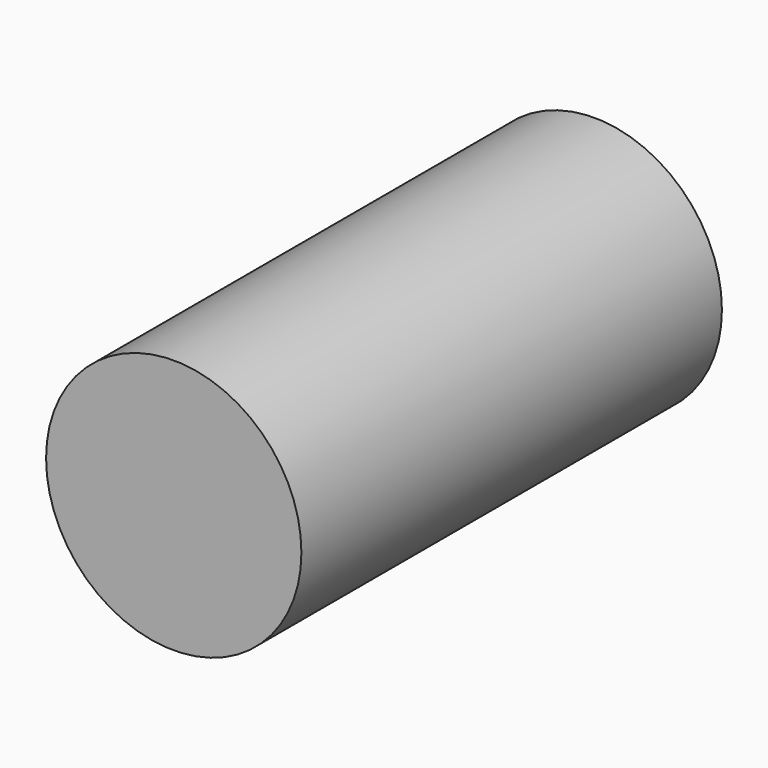
from build123d import *

# Parameters (mm, degrees)
F1_R     = 37.0145750202
F2_DEPTH = 152.4


# Not quite as in the source:
# - the program builds the solid bodies; features that only make, move or delete a surface that nothing else refers to are left out


with BuildPart() as f2:
    # F1 (on face) → F2 (new body)
    with BuildSketch(Plane.XZ):
        Circle(F1_R)
    extrude(amount=F2_DEPTH)


solid = f2.part
